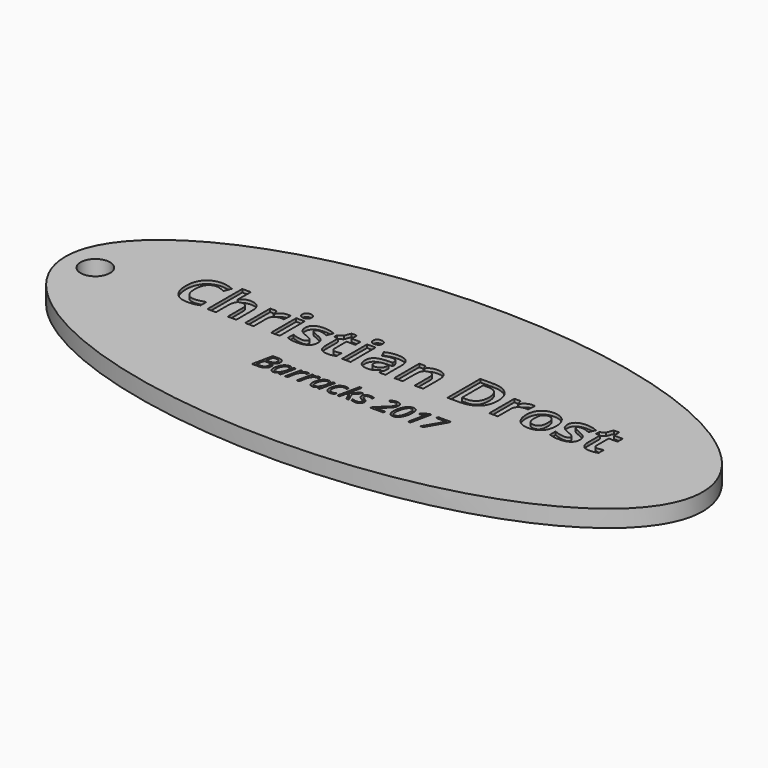
from build123d import *

# Parameters (mm, degrees)
F1_DEPTH     = 2.032
F2_R         = 1.7519130608
F3_DEPTH     = 21.336
F4_TEXT_SIZE = 6.829970813
F5_DEPTH     = 0.381
F6_TEXT_SIZE = 3.4352989225
F7_DEPTH     = 1.27


# Not quite as in the source:
# - Text() gives the source's letters only with a copy of the font that has no kerning and outlines rounded to 1/6400 em; it was checked with that copy


with BuildPart() as f1:
    # F0 (on Top) → F1 (new body)
    with BuildSketch(Plane.XY):
        with BuildLine():
            add(Edge.make_bspline(
                [(-37.9414968193, 0), (-37.9414968193, -29.0004525449), (18.9707484096, -14.5002262724), (75.8829936385, 0), (18.9707484096, 14.5002262724), (-37.9414968193, 29.0004525449), (-37.9414968193, 0)],
                knots=[0, 0, 0, 2.0943951024, 2.0943951024, 4.1887902048, 4.1887902048, 6.2831853072, 6.2831853072, 6.2831853072], degree=2, weights=[1, 0.5, 1, 0.5, 1, 0.5, 1]))
        make_face()
    extrude(amount=F1_DEPTH)

    # F2 (on face) → F3 (cut)
    with BuildSketch(Plane.XY.offset(2.032)):
        with Locations((-34.373331815, 0)):
            Circle(F2_R)
    extrude(amount=-F3_DEPTH, mode=Mode.SUBTRACT)

    # F4 (on face) → F5 (cut)
    with BuildSketch(Plane.XY.offset(2.032)):
        with Locations((-25.9138697293, 0)):
            Text('Christian Drost', F4_TEXT_SIZE, font='Open Sans', font_style=FontStyle.BOLD, text_align=(TextAlign.LEFT, TextAlign.BOTTOM))
    extrude(amount=-F5_DEPTH, mode=Mode.SUBTRACT)

    # F6 (on face) → F7 (cut)
    with BuildSketch(Plane.XY.offset(2.032)):
        with Locations((-11.031335282, -6.0444067357)):
            Text('Barracks 2017', F6_TEXT_SIZE, font='Open Sans', font_style=FontStyle.ITALIC, text_align=(TextAlign.LEFT, TextAlign.BOTTOM))
    extrude(amount=-F7_DEPTH, mode=Mode.SUBTRACT)


solid = f1.part
